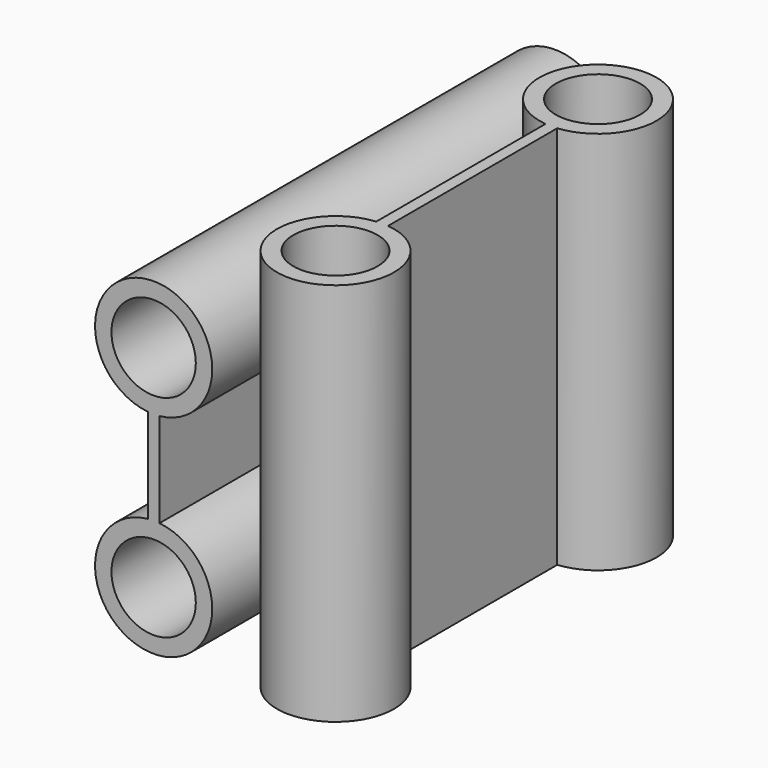
from build123d import *

# Parameters (mm, degrees)
F2_DEPTH      = 107
F2_DEPTH_BACK = 107
F0_R          = 18
F3_DEPTH      = 107
F3_DEPTH_BACK = 107
F1_R          = 18
F4_DEPTH      = 82
F4_DEPTH_BACK = 82


# Not quite as in the source:
# - a feature of the source that left no trace in its solid (it failed there, or was rolled back) is left out


with BuildPart() as f2:
    # F0 (on Front) → F2 (new body, two sides)
    with BuildSketch(Plane.XZ) as f2_sk:
        with BuildLine():
            ThreePointArc((-45.5, 20.1253140723), (-48, 20), (-50.5, 20.1253140723))
            Line((-50.5, 20.1253140723), (-50.5, -20.1253140723))
            ThreePointArc((-50.5, -20.1253140723), (-48, -20), (-45.5, -20.1253140723))
            Line((-45.5, -20.1253140723), (-45.5, 20.1253140723))
        make_face()
        with BuildLine():
            Line((-45.5, 20.1253140723), (-50.5, 20.1253140723))
            ThreePointArc((-50.5, 20.1253140723), (-48, 20), (-45.5, 20.1253140723))
        make_face()
        with BuildLine():
            ThreePointArc((-45.5, -20.1253140723), (-48, -20), (-50.5, -20.1253140723))
            Line((-50.5, -20.1253140723), (-45.5, -20.1253140723))
        make_face()
    extrude(amount=F2_DEPTH)
    extrude(f2_sk.sketch, amount=-F2_DEPTH_BACK)

    # F0 (on Front) → F3 (join, two sides)
    with BuildSketch(Plane.XZ) as f3_sk:
        with BuildLine():
            ThreePointArc((-45.5, 20.1253140723), (-29.4595037823, 28.2294901688), (-23, 45))
            ThreePointArc((-23, 45), (-64.7705098312, 63.5404962177), (-50.5, 20.1253140723))
            Line((-50.5, 20.1253140723), (-45.5, 20.1253140723))
        make_face()
        with Locations((-48, 45)):
            Circle(F0_R, mode=Mode.SUBTRACT)
        with BuildLine():
            Line((-45.5, -20.1253140723), (-50.5, -20.1253140723))
            ThreePointArc((-50.5, -20.1253140723), (-64.7705098312, -63.5404962177), (-23, -45))
            ThreePointArc((-23, -45), (-29.4595037823, -28.2294901688), (-45.5, -20.1253140723))
        make_face()
        with Locations((-48, -45)):
            Circle(F0_R, mode=Mode.SUBTRACT)
    extrude(amount=F3_DEPTH)
    extrude(f3_sk.sketch, amount=-F3_DEPTH_BACK)

    # F1 (on Top) → F4 (join, two sides)
    with BuildSketch(Plane.XY) as f4_sk:
        with BuildLine():
            ThreePointArc((2.5, 45.1253140723), (18.5404962177, 53.2294901688), (25, 70))
            ThreePointArc((25, 70), (-16.7705098312, 88.5404962177), (-2.5, 45.1253140723))
            Line((-2.5, 45.1253140723), (2.5, 45.1253140723))
        make_face()
        with Locations((0, 70)):
            Circle(F1_R, mode=Mode.SUBTRACT)
        with BuildLine():
            Line((2.5, 45.1253140723), (-2.5, 45.1253140723))
            ThreePointArc((-2.5, 45.1253140723), (0, 45), (2.5, 45.1253140723))
        make_face()
        with BuildLine():
            ThreePointArc((2.5, 45.1253140723), (0, 45), (-2.5, 45.1253140723))
            Line((-2.5, 45.1253140723), (-2.5, -45.1253140723))
            ThreePointArc((-2.5, -45.1253140723), (0, -45), (2.5, -45.1253140723))
            Line((2.5, -45.1253140723), (2.5, 45.1253140723))
        make_face()
        with BuildLine():
            ThreePointArc((2.5, -45.1253140723), (0, -45), (-2.5, -45.1253140723))
            Line((-2.5, -45.1253140723), (2.5, -45.1253140723))
        make_face()
        with BuildLine():
            Line((2.5, -45.1253140723), (-2.5, -45.1253140723))
            ThreePointArc((-2.5, -45.1253140723), (-16.7705098312, -88.5404962177), (25, -70))
            ThreePointArc((25, -70), (18.5404962177, -53.2294901688), (2.5, -45.1253140723))
        make_face()
        with Locations((0, -70)):
            Circle(F1_R, mode=Mode.SUBTRACT)
    extrude(amount=F4_DEPTH)
    extrude(f4_sk.sketch, amount=-F4_DEPTH_BACK)


solid = f2.part
